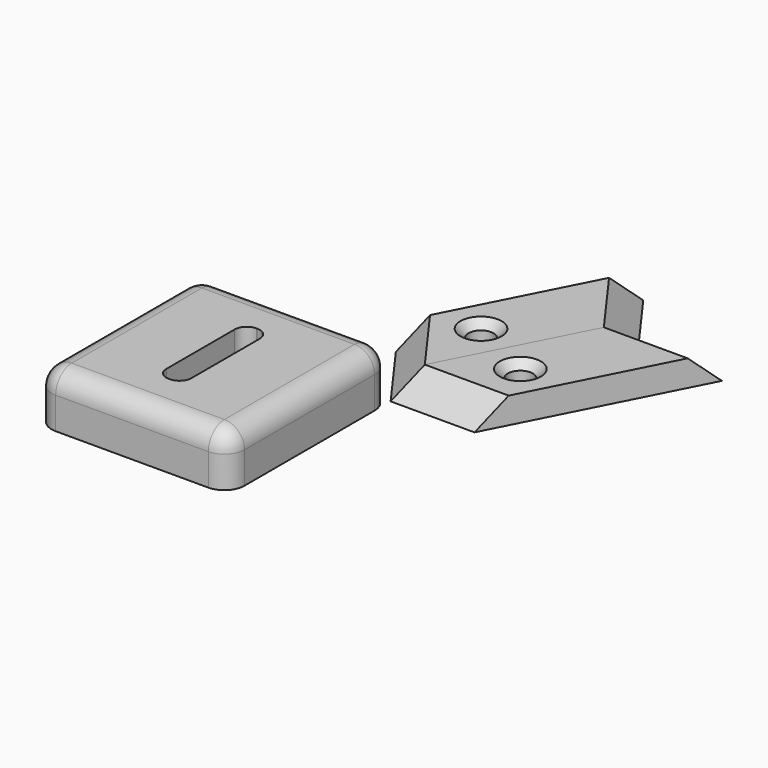
from build123d import *

# Parameters (mm, degrees)
F1_DEPTH = 12.9
F2_R     = 5
F3_R     = 3.125
F4_DEPTH = 6.5
F5_SIZE  = 6.49999
F6_SIZE  = 2


# Not quite as in the source:
# - a fillet or chamfer is up to 0.001 mm smaller than in the source, because OpenCascade refuses the exact size


with BuildPart() as f1:
    # F0 (on Top) → F1 (new body)
    with BuildSketch(Plane.XY):
        with BuildLine():
            ThreePointArc((-48, -45.5), (-46.5355339059, -49.0355339059), (-43, -50.5))
            Line((-43, -50.5), (-5, -50.5))
            ThreePointArc((-5, -50.5), (-1.4644660941, -49.0355339059), (0, -45.5))
            Line((0, -45.5), (0, -5))
            ThreePointArc((0, -5), (-1.4644660941, -1.4644660941), (-5, 0))
            Line((-5, 0), (-43, 0))
            ThreePointArc((-43, 0), (-46.5355339059, -1.4644660941), (-48, -5))
            Line((-48, -5), (-48, -45.5))
        make_face()
        with BuildLine():
            ThreePointArc((-27.125, -14.625), (-26.2463203436, -12.5036796564), (-24.125, -11.625))
            Line((-24.125, -11.625), (-23.875, -11.625))
            ThreePointArc((-23.875, -11.625), (-21.7536796564, -12.5036796564), (-20.875, -14.625))
            Line((-20.875, -14.625), (-20.875, -35.875))
            ThreePointArc((-20.875, -35.875), (-21.7536796564, -37.9963203436), (-23.875, -38.875))
            Line((-23.875, -38.875), (-24.125, -38.875))
            ThreePointArc((-24.125, -38.875), (-26.2463203436, -37.9963203436), (-27.125, -35.875))
            Line((-27.125, -35.875), (-27.125, -14.625))
        make_face(mode=Mode.SUBTRACT)
    extrude(amount=F1_DEPTH)

    # F2
    f2_edges = [f1.edges().sort_by_distance(p)[0] for p in [
        (0, -25.25, 12.9),
        (-1.464466, -49.035534, 12.9),
        (-24, -50.5, 12.9),
        (-46.535534, -49.035534, 12.9),
        (-48, -25.25, 12.9),
        (-46.535534, -1.464466, 12.9),
        (-24, 0, 12.9),
        (-1.464466, -1.464466, 12.9),
    ]]
    fillet(f2_edges, radius=F2_R)


with BuildPart() as f4:
    # F3 (on Top) → F4 (new body)
    with BuildSketch(Plane.XY):
        Polygon((24.0128942012, 47), (0, 0), (20.8869944401, 0), (44.8998886413, 47), align=None)
        with Locations((18.9628277648, 16.6747303447)):
            Circle(F3_R, mode=Mode.SUBTRACT)
    extrude(amount=F4_DEPTH)

    # F5 (size 6.5 in the source; OpenCascade refuses exactly that, so slightly less here)
    f5_edges = [f4.edges().sort_by_distance(p)[0] for p in [
        (10.443497, 0, 6.5),
        (34.456391, 47, 6.5),
    ]]
    chamfer(f5_edges, length=F5_SIZE)

    # F6
    f6_edges = [f4.edges().sort_by_distance(p)[0] for p in [
        (15.837828, 16.67473, 6.5),
    ]]
    chamfer(f6_edges, length=F6_SIZE)


with BuildPart() as f7_1:
    # F7: instance of F4
    add(f4.part.mirror(Plane(origin=(12.0064471006, 23.5, 3.0761317731), x_dir=(-0.4549709236, -0.8905062934, 0), z_dir=(-0.8905062934, 0.4549709236, 0))))


solid = Compound([f1.part, f4.part, f7_1.part])
